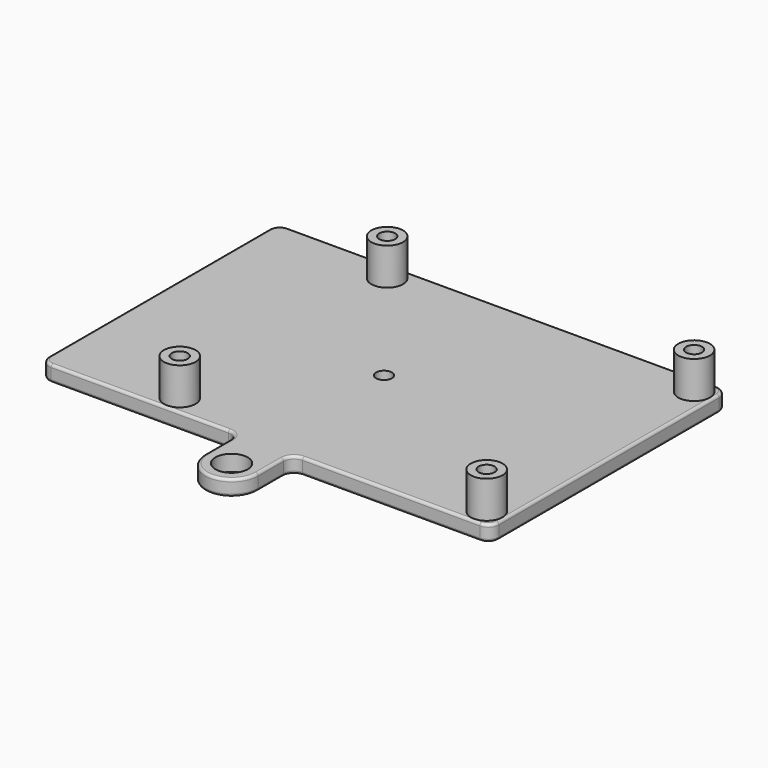
from build123d import *

# Parameters (mm, degrees)
F0_R     = 3
F0_R_2   = 3.05
F0_R_3   = 1.5
F1_DEPTH = 3
F2_DEPTH = 10
F3_R     = 0.49999


# Not quite as in the source:
# - a fillet or chamfer is up to 0.001 mm smaller than in the source, because OpenCascade refuses the exact size
# - a feature names something its author has since deleted; it is built from what else it names


with BuildPart() as f1:
    # F0 (on Top) → F1 (new body)
    with BuildSketch(Plane.XY):
        with BuildLine():
            ThreePointArc((42.5, 26), (41.9142135624, 27.4142135624), (40.5, 28))
            Line((40.5, 28), (-40.5, 28))
            ThreePointArc((-40.5, 28), (-41.9142135624, 27.4142135624), (-42.5, 26))
            Line((-42.5, 26), (-42.5, -26))
            ThreePointArc((-42.5, -26), (-41.9142135624, -27.4142135624), (-40.5, -28))
            Line((-40.5, -28), (-7, -28))
            ThreePointArc((-7, -28), (-5.5857864376, -28.5857864376), (-5, -30))
            Line((-5, -30), (-5, -36))
            ThreePointArc((-5, -36), (0, -41), (5, -36))
            Line((5, -36), (5, -30))
            ThreePointArc((5, -30), (5.5857864376, -28.5857864376), (7, -28))
            Line((7, -28), (40.5, -28))
            ThreePointArc((40.5, -28), (41.9142135624, -27.4142135624), (42.5, -26))
            Line((42.5, -26), (42.5, 26))
        make_face()
        with Locations((-19, -24.5)):
            Circle(F0_R, mode=Mode.SUBTRACT)
        with Locations((0, -36)):
            Circle(F0_R_2, mode=Mode.SUBTRACT)
        with Locations((39, -24.5)):
            Circle(F0_R, mode=Mode.SUBTRACT)
        with Locations((-19, 24.5)):
            Circle(F0_R, mode=Mode.SUBTRACT)
        Circle(F0_R_3, mode=Mode.SUBTRACT)
        with Locations((39, 24.5)):
            Circle(F0_R, mode=Mode.SUBTRACT)
    extrude(amount=F1_DEPTH)

    # F0 (on Top) → F2 (join)
    with BuildSketch(Plane.XY):
        with Locations((-19, -24.5)):
            Circle(F0_R)
        with Locations((-19, -24.5)):
            Circle(F0_R_3, mode=Mode.SUBTRACT)
        with Locations((-19, 24.5)):
            Circle(F0_R)
        with Locations((-19, 24.5)):
            Circle(F0_R_3, mode=Mode.SUBTRACT)
        with Locations((39, 24.5)):
            Circle(F0_R)
        with Locations((39, 24.5)):
            Circle(F0_R_3, mode=Mode.SUBTRACT)
        with Locations((39, -24.5)):
            Circle(F0_R)
        with Locations((39, -24.5)):
            Circle(F0_R_3, mode=Mode.SUBTRACT)
    extrude(amount=F2_DEPTH)

    # F3 (radius 0.5 in the source; OpenCascade refuses exactly that, so slightly less here)
    f3_edges = [f1.edges().sort_by_distance(p)[0] for p in [
        (23.75, -28, 3),
        (23.75, -28, 0),
    ]]
    fillet(f3_edges, radius=F3_R)


solid = f1.part
